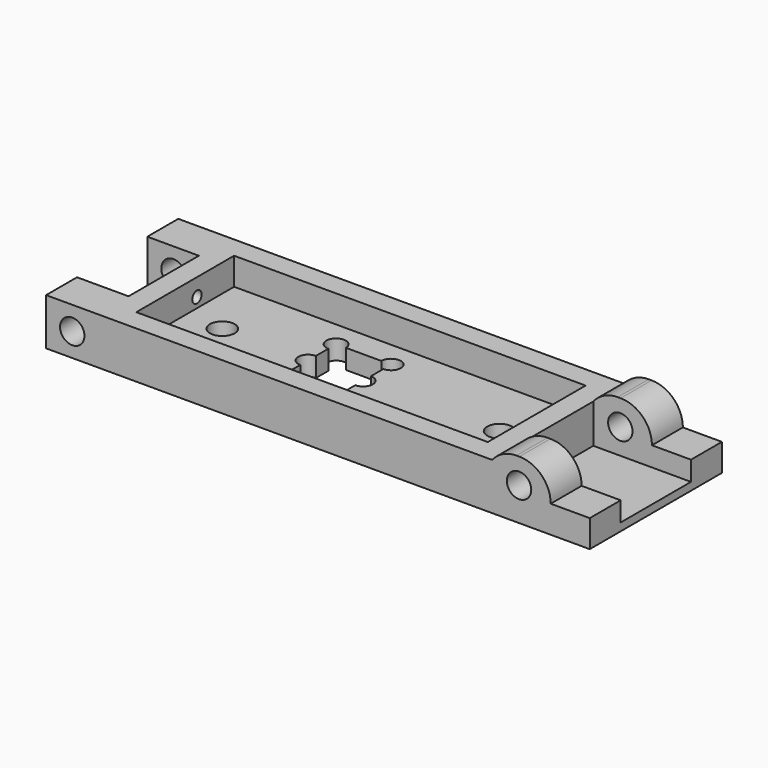
from build123d import *

# Parameters (mm, degrees)
F0_W         = 3.3528
F0_H         = 2.5146
F0_R         = 0.80645
F0_W_2       = 6.35
F0_H_2       = 10.7442
F1_DEPTH     = 3.048
F2_W         = 2.54
F2_H         = 10.7442
F2_W_2       = 22.86
F2_H_2       = 7.9502
F3_DEPTH     = 1.27
F4_W         = 6.35
F4_H         = 5.715
F5_DEPTH     = 2.54
F6_R         = 0.79375
F7_DEPTH     = 10.7452
F8_DEPTH     = 0.508
F9_W         = 3.81
F9_H         = 2.5146
F10_DEPTH    = 0.762
F11_T1_DEPTH = 10.445747458
F11_T3_DEPTH = 10.445747458
F11_T5_DEPTH = 12.6746
F11_T7_DEPTH = 12.6746
F12_R        = 0.381
F13_DEPTH    = 1.397


# Not quite as in the source:
# - a fillet or chamfer that OpenCascade refuses, or shapes differently, is made with other operations: its cross-section is extruded or revolved along the edge and cut away or added
# - a feature names something its author has since deleted; it is built from what else it names


with BuildPart() as f1:
    # F0 (on Top) → F1 (new body)
    with BuildSketch(Plane.XY):
        with Locations((-12.8524, 4.1148)):
            Rectangle(F0_W, F0_H)
        with Locations((-12.8524, -4.1148)):
            Rectangle(F0_W, F0_H)
        Polygon((14.478, -5.3721), (14.478, 5.3721), (-11.176, 5.3721), (-11.176, 2.8575), (-11.176, -2.8575), (-11.176, -5.3721), align=None)
        with Locations((-7.366, 0)):
            Circle(F0_R, mode=Mode.SUBTRACT)
        with BuildLine():
            ThreePointArc((-1.7885716042, 1.644670926), (-2.2375844102, 2.728683732), (-1.1535716042, 2.279670926))
            Line((-1.1535716042, 2.279670926), (1.1535716042, 2.279670926))
            ThreePointArc((1.1535716042, 2.279670926), (2.2375844102, 2.728683732), (1.7885716042, 1.644670926))
            Line((1.7885716042, 1.644670926), (1.7885716042, 0.635))
            ThreePointArc((1.7885716042, 0.635), (2.4235716042, 0), (1.7885716042, -0.635))
            Line((1.7885716042, -0.635), (1.7885716042, -1.644670926))
            ThreePointArc((1.7885716042, -1.644670926), (2.2375844102, -2.728683732), (1.1535716042, -2.279670926))
            Line((1.1535716042, -2.279670926), (-1.1535716042, -2.279670926))
            ThreePointArc((-1.1535716042, -2.279670926), (-2.2375844102, -2.728683732), (-1.7885716042, -1.644670926))
            Line((-1.7885716042, -1.644670926), (-1.7885716042, -0.635))
            ThreePointArc((-1.7885716042, -0.635), (-2.4235716042, 0), (-1.7885716042, 0.635))
            Line((-1.7885716042, 0.635), (-1.7885716042, 1.644670926))
        make_face(mode=Mode.SUBTRACT)
        with Locations((10.668, 0)):
            Circle(F0_R, mode=Mode.SUBTRACT)
        with Locations((17.653, 0)):
            Rectangle(F0_W_2, F0_H_2)
    extrude(amount=F1_DEPTH)

    # F2 (on face) → F3 (cut)
    with BuildSketch(Plane.XY.offset(3.048)):
        with Locations((19.558, 0)):
            Rectangle(F2_W, F2_H)
        with Locations((1.651, 0)):
            Rectangle(F2_W_2, F2_H_2)
    extrude(amount=-F3_DEPTH, mode=Mode.SUBTRACT)

    # F4 (on face) → F5 (cut)
    with BuildSketch(Plane.XY.offset(3.048)):
        with Locations((17.653, 0)):
            Rectangle(F4_W, F4_H)
    extrude(amount=-F5_DEPTH, mode=Mode.SUBTRACT)

    # F6 (on face) → F7 (cut, through all)
    with BuildSketch(Plane.XZ.offset(5.3721)):
        with Locations((-12.827, 1.524)):
            Circle(F6_R)
        with Locations((16.2306, 2.159)):
            Circle(F6_R)
    extrude(amount=-F7_DEPTH, mode=Mode.SUBTRACT)

    # F8 (cut): a face of the model
    f8_faces = [f1.faces().sort_by_distance(p)[0] for p in [
        (-9.5369699853, 0, 1.778),
    ]]
    extrude(f8_faces, amount=-F8_DEPTH, mode=Mode.SUBTRACT)

    # F9 (on face) → F10 (join)
    with BuildSketch(Plane.XY.offset(3.048)):
        with Locations((16.383, 4.1148)):
            Rectangle(F9_W, F9_H)
        with Locations((16.383, -4.1148)):
            Rectangle(F9_W, F9_H)
    extrude(amount=F10_DEPTH)

    # F11: fillet of radius 2.032 on 4 edges, made by hand

    # F11_s2 → F11_t1 (cut)
    with BuildSketch(Plane.XZ.offset(-1.108073729)):
        with BuildLine():
            ThreePointArc((16.0642294916, 3.81), (15.1843476813, 3.6096200479), (14.478, 3.048))
            Line((14.478, 3.048), (14.478, 3.81))
            Line((14.478, 3.81), (16.0642294916, 3.81))
        make_face()
    extrude(amount=F11_T1_DEPTH, mode=Mode.SUBTRACT)

    # F11_s4 → F11_t3 (cut)
    with BuildSketch(Plane.XZ.offset(-9.337673729)):
        with BuildLine():
            ThreePointArc((16.0642294916, 3.81), (15.1843476813, 3.6096200479), (14.478, 3.048))
            Line((14.478, 3.048), (14.478, 3.81))
            Line((14.478, 3.81), (16.0642294916, 3.81))
        make_face()
    extrude(amount=F11_T3_DEPTH, mode=Mode.SUBTRACT)

    # F11_s6 → F11_t5 (cut)
    with BuildSketch(Plane.XZ.offset(-10.4521)):
        with BuildLine():
            ThreePointArc((18.288, 1.778), (17.6928409794, 3.2148409794), (16.256, 3.81))
            Line((16.256, 3.81), (18.288, 3.81))
            Line((18.288, 3.81), (18.288, 1.778))
        make_face()
    extrude(amount=F11_T5_DEPTH, mode=Mode.SUBTRACT)

    # F11_s8 → F11_t7 (cut)
    with BuildSketch(Plane.XZ.offset(-2.2225)):
        with BuildLine():
            ThreePointArc((18.288, 1.778), (17.6928409794, 3.2148409794), (16.256, 3.81))
            Line((16.256, 3.81), (18.288, 3.81))
            Line((18.288, 3.81), (18.288, 1.778))
        make_face()
    extrude(amount=F11_T7_DEPTH, mode=Mode.SUBTRACT)

    # F12 (on face) → F13 (cut, through all)
    with BuildSketch(Plane(origin=(-11.176, 0, 0), x_dir=(0, -1, 0), z_dir=(-1, 0, 0))):
        with Locations((-0.9525, 1.9129452994)):
            Circle(F12_R)
    extrude(amount=-F13_DEPTH, mode=Mode.SUBTRACT)


solid = f1.part
